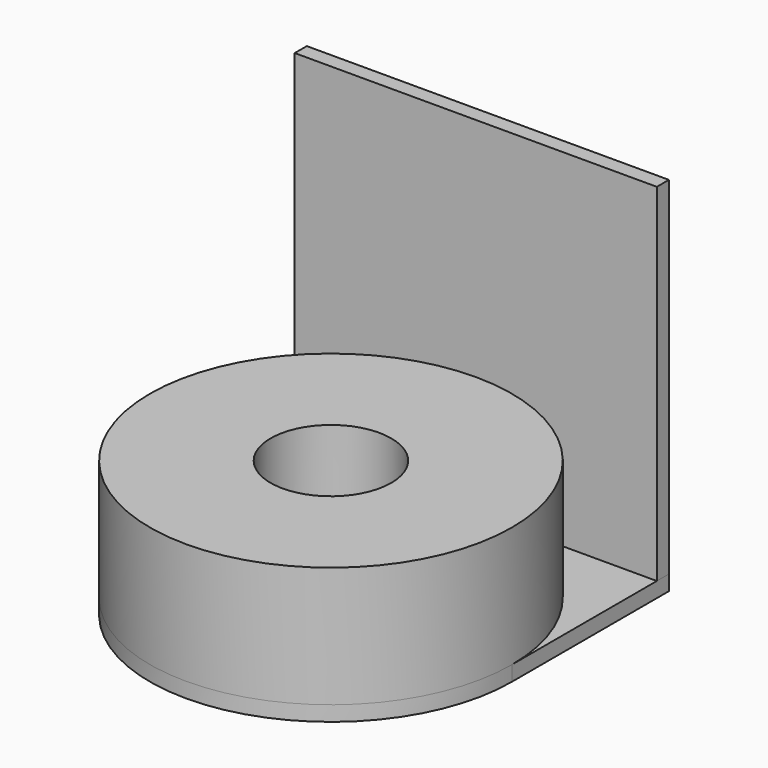
from build123d import *

# Parameters (mm, degrees)
F1_DEPTH = 25.4
F0_R     = 12.7
F2_DEPTH = 3.175
F3_DEPTH = 47.625


with BuildPart() as f1:
    # F0 (on Top) → F1 (new body)
    with BuildSketch(Plane.XY):
        Polygon((-38.1, 38.1), (0, 38.1), (38.1, 38.1), (38.1, 41.275), (-38.1, 41.275), align=None)
    extrude(amount=F1_DEPTH)

    # F3 (add): a face of the model
    f3_faces = [f1.faces().sort_by_distance(p)[0] for p in [
        (0, 39.6875, 25.4),
    ]]
    extrude(f3_faces, amount=F3_DEPTH)


with BuildPart() as f1b:
    # F0 (on Top) → F1, piece 2 (new body)
    with BuildSketch(Plane.XY):
        with BuildLine():
            ThreePointArc((0, 38.1), (-26.9407683632, 26.9407683632), (-38.1, 0))
            ThreePointArc((-38.1, 0), (0, -38.1), (38.1, 0))
            ThreePointArc((38.1, 0), (26.9407683632, 26.9407683632), (0, 38.1))
        make_face()
        Circle(F0_R, mode=Mode.SUBTRACT)
    extrude(amount=F1_DEPTH)

    # F0 (on Top) → F2 (join)
    with BuildSketch(Plane.XY):
        with BuildLine():
            ThreePointArc((0, 38.1), (26.9407683632, 26.9407683632), (38.1, 0))
            Line((38.1, 0), (38.1, 38.1))
            Line((38.1, 38.1), (0, 38.1))
        make_face()
        with BuildLine():
            Line((-38.1, 38.1), (-38.1, 0))
            ThreePointArc((-38.1, 0), (-26.9407683632, 26.9407683632), (0, 38.1))
            Line((0, 38.1), (-38.1, 38.1))
        make_face()
        Polygon((-38.1, 38.1), (0, 38.1), (38.1, 38.1), (38.1, 41.275), (-38.1, 41.275), align=None)
        with BuildLine():
            ThreePointArc((0, 38.1), (-26.9407683632, 26.9407683632), (-38.1, 0))
            ThreePointArc((-38.1, 0), (0, -38.1), (38.1, 0))
            ThreePointArc((38.1, 0), (26.9407683632, 26.9407683632), (0, 38.1))
        make_face()
        Circle(F0_R, mode=Mode.SUBTRACT)
        Circle(F0_R)
    extrude(amount=-F2_DEPTH)


solid = Compound([f1.part, f1b.part])
